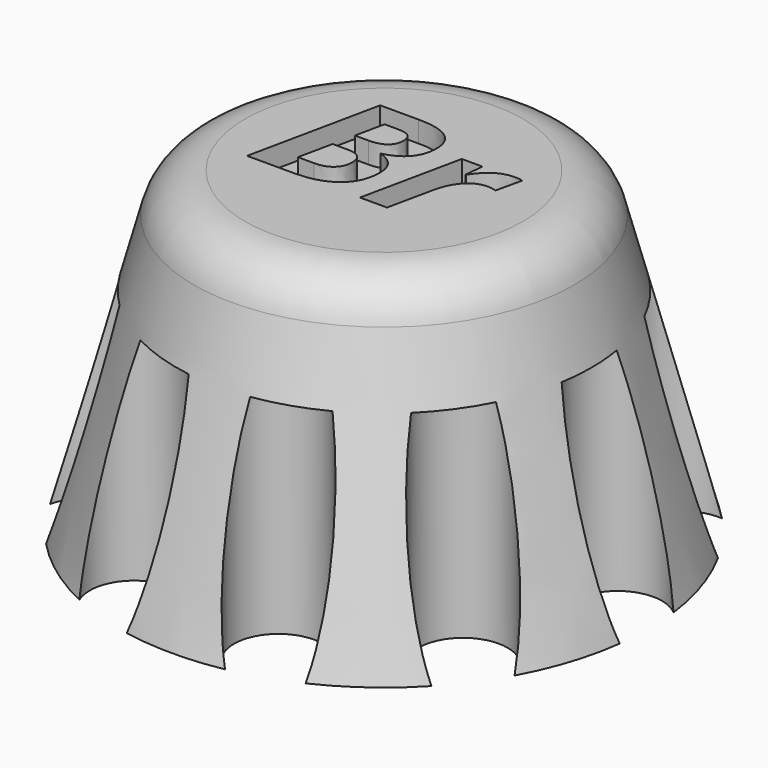
from build123d import *

# Parameters (mm, degrees)
F0_R         = 25
F1_DEPTH     = 30
F1_TAPER     = 15
F3_DEPTH     = 20
F5_R         = 5
F4_R         = 4.206085498
F6_DEPTH     = 20
F7_TEXT_SIZE = 17.4096766083
F8_DEPTH     = 2


# Not quite as in the source:
# - Text() gives the source's letters only with a copy of the font that has no kerning and outlines rounded to 1/6400 em; it was checked with that copy


with BuildPart() as f1:
    # F0 (on Top) → F1 (new body)
    with BuildSketch(Plane.XY):
        Circle(F0_R)
    extrude(amount=F1_DEPTH, taper=F1_TAPER)

    # F2 (on Top) → F3 (cut)
    with BuildSketch(Plane.XY):
        with BuildLine():
            Line((-1.1280539911, 2.2310298503), (-1.1280539911, -2.2310298503))
            ThreePointArc((-1.1280539911, -2.2310298503), (2.5, 0), (-1.1280539911, 2.2310298503))
        make_face()
    extrude(amount=F3_DEPTH, mode=Mode.SUBTRACT)

    # F5
    f5_edges = [f1.edges().sort_by_distance(p)[0] for p in [
        (-16.961524, 0, 30),
    ]]
    fillet(f5_edges, radius=F5_R)

    # F4 (on Top) → F6 (cut)
    with BuildSketch(Plane.XY):
        with Locations((22.0432637906, 0)):
            Circle(F4_R)
        with Locations((17.8333750181, 12.9567053685)):
            Circle(F4_R)
        with Locations((6.8117431228, 20.9643896685)):
            Circle(F4_R)
        with Locations((-6.8117431228, 20.9643896685)):
            Circle(F4_R)
        with Locations((-17.8333750181, 12.9567053685)):
            Circle(F4_R)
        with Locations((-22.0432637906, 0)):
            Circle(F4_R)
        with Locations((-17.8333750181, -12.9567053685)):
            Circle(F4_R)
        with Locations((-6.8117431228, -20.9643896685)):
            Circle(F4_R)
        with Locations((6.8117431228, -20.9643896685)):
            Circle(F4_R)
        with Locations((17.8333750181, -12.9567053685)):
            Circle(F4_R)
    extrude(amount=F6_DEPTH, mode=Mode.SUBTRACT)

    # F7 (on face) → F8 (cut)
    with BuildSketch(Plane.XY.offset(30)):
        with Locations((-9.768744465, -4.5176672866)):
            Text('Br', F7_TEXT_SIZE, font='Open Sans', font_style=FontStyle.BOLDITALIC, text_align=(TextAlign.LEFT, TextAlign.BOTTOM))
    extrude(amount=-F8_DEPTH, mode=Mode.SUBTRACT)


solid = f1.part
